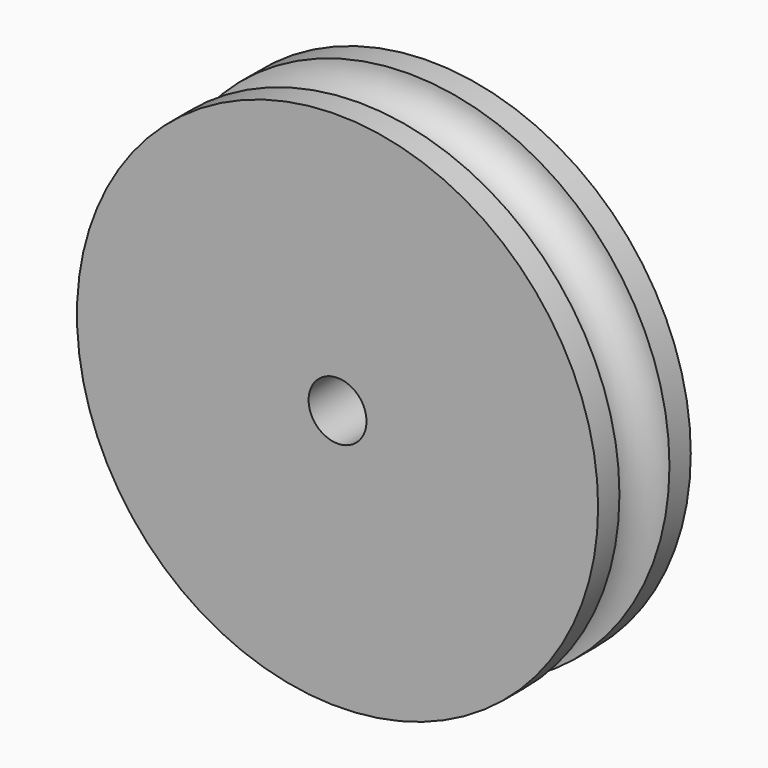
from build123d import *

# Parameters (mm, degrees)
F1_R     = 31.75
F2_DEPTH = 7.0555555556
F5_R     = 3.5277777778
F6_DEPTH = 14.1111111111


# Not quite as in the source:
# - a variable given as a bare number and used for a length is read in inches; the dataset says mm whatever the document's units were


with BuildPart() as f2:
    # F1 (on Front) → F2 (new body, symmetric)
    with BuildSketch(Plane.XZ):
        Circle(F1_R)
    extrude(amount=F2_DEPTH, both=True)

    # F3 (on Right) → F4 (revolve, cut)
    with BuildSketch(Plane.YZ):
        with BuildLine():
            Line((3.81, 31.75), (-3.81, 31.75))
            ThreePointArc((-3.81, 31.75), (0, 27.94), (3.81, 31.75))
        make_face()
    revolve(axis=Axis((0, -7.0555555556, 0), (0, -1, 0)), mode=Mode.SUBTRACT)

    # F5 (on face) → F6 (cut, through all)
    with BuildSketch(Plane(origin=(0, 7.0555555556, 0), x_dir=(-1, 0, 0), z_dir=(0, 1, 0))):
        Circle(F5_R)
    extrude(amount=-F6_DEPTH, mode=Mode.SUBTRACT)


solid = f2.part
